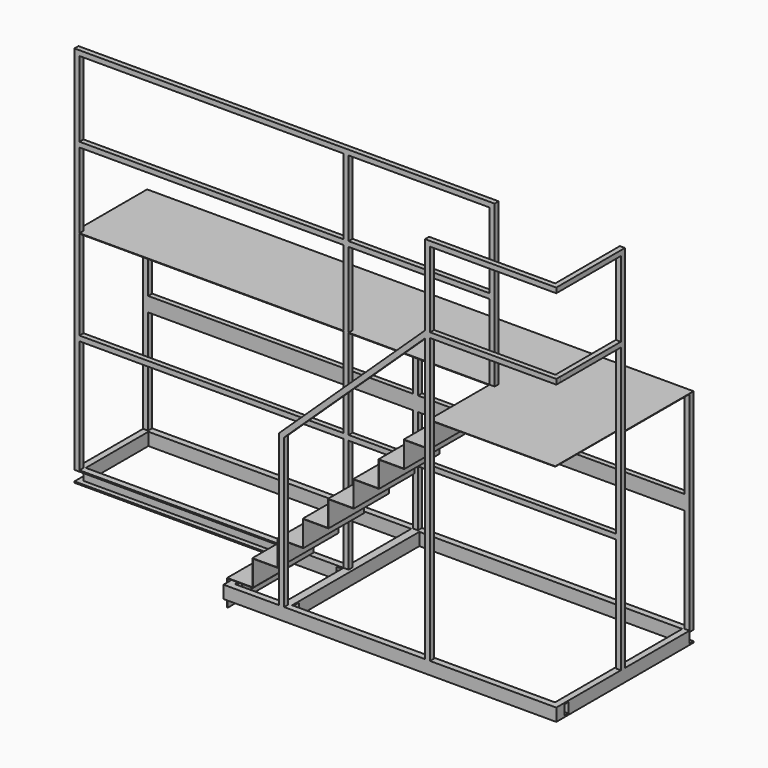
from build123d import *

# Parameters (mm, degrees)
F0_W          = 2082.9370811584
F0_H          = 620
F0_W_2        = 50
F0_H_2        = 590
F1_DEPTH      = 100
F2_W          = 40
F2_H          = 80
F3_DEPTH      = 1692.9370811584
F4_DEPTH      = 4330.001
F5_W          = 40
F5_H          = 80
F6_DEPTH      = 680.001
F8_W          = 90
F8_H          = 80
F9_DEPTH      = 630
F9_DEPTH_BACK = 70
F10_W         = 40
F10_H         = 40
F11_DEPTH     = 2930
F12_W         = 4330
F12_H         = 720
F13_DEPTH     = 4
F14_DEPTH     = 1650
F15_W         = 40
F15_H         = 40
F15_H_2       = 115
F16_DEPTH     = 4300
F20_DEPTH     = 600
F21_W         = 40
F21_H         = 40
F22_DEPTH     = 2930
F23_DEPTH     = 1200
F24_W         = 1000.3309154511
F24_H         = 40
F24_W_2       = 1000
F25_DEPTH     = 40
F17_W         = 40
F17_H         = 40
F26_DEPTH     = 610
F27_W         = 40
F27_H         = 40
F28_DEPTH     = 1275
F29_W         = 960
F29_H         = 1083.7077188492
F30_DEPTH     = 50
F31_W         = 40
F31_H         = 80
F32_DEPTH     = 2637


# Not quite as in the source:
# - a feature names something its author has since deleted; it is built from what else it names


with BuildPart() as f1:
    # F0 (on Top) → F1 (new body)
    with BuildSketch(Plane.XY):
        Polygon((2165, -680), (2165, 680), (-2165, 680), (-2165, -40), (-472.0629188416, -40), (-422.0629188416, -40), (-32.0629188416, -40), (-32.0629188416, -630), (-32.0629188416, -680), align=None)
        with Locations((-1073.5314594208, 320)):
            Rectangle(F0_W, F0_H, mode=Mode.SUBTRACT)
        Polygon((2115, 630), (2115, -630), (32.0629188416, -630), (32.0629188416, -9.9903011755), (32.0629188416, 630), align=None, mode=Mode.SUBTRACT)
        with Locations((-447.0629188416, -335)):
            Rectangle(F0_W_2, F0_H_2)
        Polygon((-472.0629188416, -680), (-32.0629188416, -680), (-32.0629188416, -630), (-422.0629188416, -630), (-472.0629188416, -630), align=None)
    extrude(amount=F1_DEPTH)

    # F2 (on face) → F3 (cut, through all)
    with BuildSketch(Plane(origin=(-2165, 0, 0), x_dir=(0, -1, 0), z_dir=(-1, 0, 0))):
        with Locations((20, 50)):
            Rectangle(F2_W, F2_H)
    extrude(amount=-F3_DEPTH, mode=Mode.SUBTRACT)

    # F2 (on face) → F4 (cut, through all)
    with BuildSketch(Plane(origin=(-2165, 0, 0), x_dir=(0, -1, 0), z_dir=(-1, 0, 0))):
        with Locations((-660, 50)):
            Rectangle(F2_W, F2_H)
    extrude(amount=-F4_DEPTH, mode=Mode.SUBTRACT)

    # F5 (on face) → F6 (cut, through all)
    with BuildSketch(Plane.XZ):
        with Locations((-2145, 50)):
            Rectangle(F5_W, F5_H)
    extrude(amount=-F6_DEPTH, mode=Mode.SUBTRACT)

    # F8 (on Front) → F9 (cut, two sides)
    with BuildSketch(Plane.XZ) as f9_sk:
        with Locations((-45, 50)):
            Rectangle(F8_W, F8_H)
    extrude(amount=-F9_DEPTH, mode=Mode.SUBTRACT)
    extrude(f9_sk.sketch, amount=F9_DEPTH_BACK, mode=Mode.SUBTRACT)

    # F10 (on face) → F11 (join)
    with BuildSketch(Plane.XY.offset(100)):
        with Locations((-2145, -20)):
            Rectangle(F10_W, F10_H)
        with Locations((-12.0629188416, -20)):
            Rectangle(F10_W, F10_H)
        with Locations((2145, -20)):
            Rectangle(F10_W, F10_H)
    extrude(amount=F11_DEPTH)

    # F12 (on offset) → F13 (join)
    with BuildSketch(Plane.XY.offset(1750)):
        with Locations((0, 320)):
            Rectangle(F12_W, F12_H)
    extrude(amount=F13_DEPTH)

    # F10 (on face) → F14 (join)
    with BuildSketch(Plane.XY.offset(100)):
        with Locations((-2145, 660)):
            Rectangle(F10_W, F10_H)
        with Locations((2145, 660)):
            Rectangle(F10_W, F10_H)
        with Locations((-7.0629188416, 660)):
            Rectangle(F10_W, F10_H)
        with Locations((-2145, -20)):
            Rectangle(F10_W, F10_H)
        with Locations((-12.0629188416, -20)):
            Rectangle(F10_W, F10_H)
        with Locations((2145, -20)):
            Rectangle(F10_W, F10_H)
    extrude(amount=F14_DEPTH)

    # F15 (on face) → F16 (join)
    with BuildSketch(Plane.YZ.offset(2165)):
        with Locations((-20, 3010)):
            Rectangle(F15_W, F15_H)
        with Locations((660, 982.5)):
            Rectangle(F15_W, F15_H_2)
        with Locations((-20, 1020)):
            Rectangle(F15_W, F15_H)
        with Locations((-20, 2372)):
            Rectangle(F15_W, F15_H)
    extrude(amount=-F16_DEPTH)

    # F19 (on offset) → F20 (join)
    with BuildSketch(Plane.XZ.offset(40)):
        Polygon((2125, 1751), (2125, 1754), (1125, 1754), (1125, 1551), (925, 1551), (925, 1348), (725, 1348), (725, 1145), (525, 1145), (525, 942), (325, 942), (325, 739), (125, 739), (125, 536), (-75, 536), (-75, 333), (-275, 333), (-275, 130), (-475, 130), (-475, -75), (-472, -78), (-472, 127), (-272, 127), (-272, 330), (-72, 330), (-72, 533), (128, 533), (128, 736), (328, 736), (328, 939), (528, 939), (528, 1142), (728, 1142), (728, 1345), (928, 1345), (928, 1548), (1128, 1548), (1128, 1751), align=None)
    extrude(amount=F20_DEPTH)

    # F21 (on face) → F22 (join)
    with BuildSketch(Plane.XY.offset(100)):
        with Locations((1145, -660)):
            Rectangle(F21_W, F21_H)
    extrude(amount=F22_DEPTH)

    # F21 (on face) → F23 (join)
    with BuildSketch(Plane.XY.offset(100)):
        with Locations((-12.0629188416, -660)):
            Rectangle(F21_W, F21_H)
    extrude(amount=F23_DEPTH)

    # F24 (on face) → F25 (join)
    with BuildSketch(Plane.XZ.offset(680)):
        Polygon((1125, 2392.7055740356), (-32.0629188416, 1300), (7.9370811584, 1300), (7.9370811584, 1282.7573162751), (1125, 2337.687742348), (1125, 2352.7055740356), align=None)
        with Locations((1665.1654577255, 2372.7055740356)):
            Rectangle(F24_W, F24_H)
        with Locations((1665, 3010)):
            Rectangle(F24_W_2, F24_H)
    extrude(amount=-F25_DEPTH)

    # F17 (on face) → F26 (join)
    with BuildSketch(Plane.XZ.offset(40)):
        with Locations((2145, 2372)):
            Rectangle(F17_W, F17_H)
        with Locations((2145, 3010)):
            Rectangle(F17_W, F17_H)
    extrude(amount=F26_DEPTH)

    # F27 (on face) → F28 (join)
    with BuildSketch(Plane.XY.offset(1754)):
        with Locations((1145, -20)):
            Rectangle(F27_W, F27_H)
    extrude(amount=F28_DEPTH)

    # F29 (on face) → F30 (cut)
    with BuildSketch(Plane(origin=(0, 0, 0), x_dir=(-1, 0, 0), z_dir=(0, 1, 0))):
        with Locations((-1645, 2488.1461405754)):
            Rectangle(F29_W, F29_H)
    extrude(amount=-F30_DEPTH, mode=Mode.SUBTRACT)

    # F31 (on face) → F32 (cut, through all)
    with BuildSketch(Plane.YZ.offset(2165)):
        with Locations((-580, 50)):
            Rectangle(F31_W, F31_H)
    extrude(amount=-F32_DEPTH, mode=Mode.SUBTRACT)


solid = f1.part
